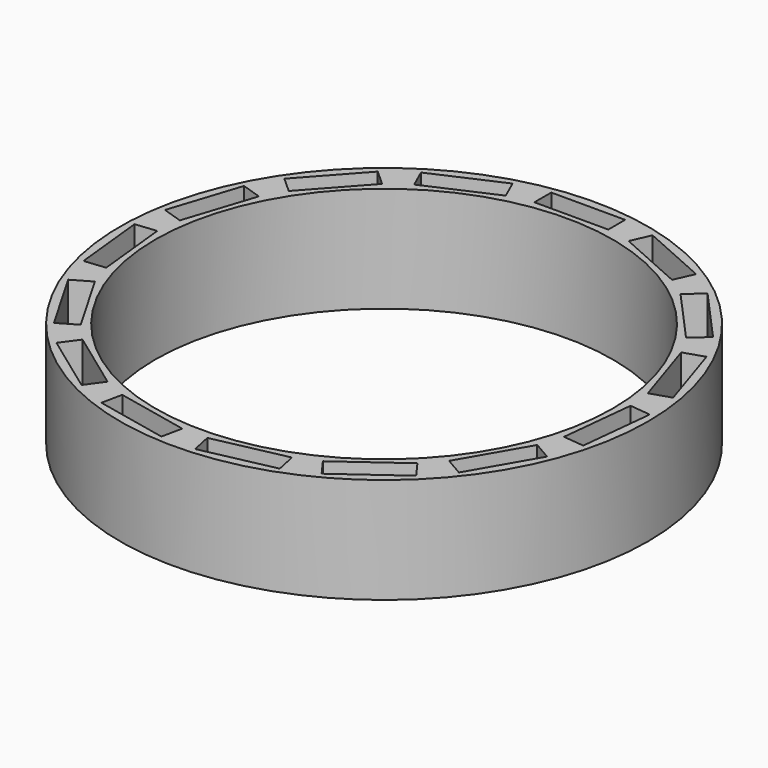
from build123d import *

# Parameters (mm, degrees)
F0_R            = 30
F0_R_2          = 26
F1_DEPTH        = 12
F2_W            = 8.4
F2_H            = 2.4
F3_DEPTH        = 11
F3_COPIES_COUNT = 15
F4_R            = 4.19999


# Not quite as in the source:
# - a fillet or chamfer is up to 0.001 mm smaller than in the source, because OpenCascade refuses the exact size
# - a pattern or mirror of a feature is missing from the dataset's text; its kind, count and spacing are read off the source's solid


with BuildPart() as f1:
    # F0 (on Top) → F1 (new body)
    with BuildSketch(Plane.XY):
        Circle(F0_R)
        Circle(F0_R_2, mode=Mode.SUBTRACT)
    extrude(amount=F1_DEPTH)

    # F2 (on face) → F3 (cut)
    with BuildSketch(Plane.XY.offset(12)):
        with Locations((0, 27.8)):
            Rectangle(F2_W, F2_H)
    f3 = extrude(amount=-F3_DEPTH, mode=Mode.SUBTRACT)

    # F3_copies: F3 ×15 about axis
    f3_copies_axis = Axis((0, 0, 0), (0, 0, 1))
    for i in range(1, F3_COPIES_COUNT):
        add(f3.rotate(f3_copies_axis, i * 360 / F3_COPIES_COUNT), mode=Mode.SUBTRACT)

    # F4 (radius 4.2 in the source; OpenCascade refuses exactly that, so slightly less here)
    f4_edges = [f1.edges().sort_by_distance(p)[0] for p in [
        (-4.2, 27.8, 1),
        (4.2, 27.8, 1),
        (-12.942559, -24.959371, 1),
        (-19.738301, -20.021974, 1),
        (-1.671725, -28.065732, 1),
        (-9.888165, -26.319274, 1),
        (-21.975506, -17.537307, 1),
        (-26.175506, -10.262693, 1),
        (-27.208689, -7.082883, 1),
        (-28.086728, 1.271101, 1),
        (9.888165, -26.319274, 1),
        (1.671725, -28.065732, 1),
        (19.738301, -20.021974, 1),
        (12.942559, -24.959371, 1),
        (26.175506, -10.262693, 1),
        (21.975506, -17.537307, 1),
        (28.086728, 1.271101, 1),
        (27.208689, -7.082883, 1),
        (-27.737243, 4.596235, 1),
        (-25.1415, 12.58511, 1),
        (-23.469775, 15.480623, 1),
        (-17.849078, 21.723039, 1),
        (-15.14417, 23.68827, 1),
        (-7.470388, 27.104858, 1),
        (25.1415, 12.58511, 1),
        (27.737243, 4.596235, 1),
        (15.14417, 23.68827, 1),
        (7.470388, 27.104858, 1),
        (17.849078, 21.723039, 1),
        (23.469775, 15.480623, 1),
    ]]
    fillet(f4_edges, radius=F4_R)


solid = f1.part
